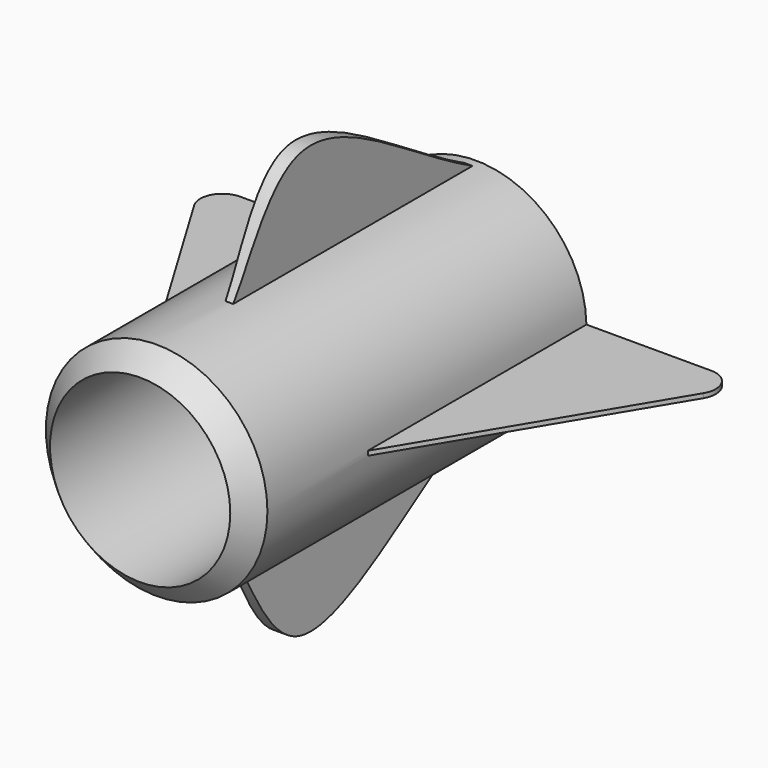
from build123d import *

# Parameters (mm, degrees)
F0_R          = 12.7
F1_DEPTH      = 50.8
F2_R          = 10.3336081204
F3_DEPTH      = 37.592
F6_DEPTH      = 0.254
F7_R          = 2.54
F9_ANGLE_BACK = 2
F9_ANGLE      = 4


# Not quite as in the source:
# - a fillet or chamfer that OpenCascade refuses, or shapes differently, is made with other operations: its cross-section is extruded or revolved along the edge and cut away or added


with BuildPart() as f1:
    # F0 (on Front) → F1 (new body)
    with BuildSketch(Plane.XZ):
        Circle(F0_R)
    extrude(amount=F1_DEPTH)

    # F2 (on face) → F3 (cut)
    with BuildSketch(Plane.XZ.offset(50.8)):
        Circle(F2_R)
    extrude(amount=-F3_DEPTH, mode=Mode.SUBTRACT)

    # F8: F6 across plane


with BuildPart() as f6:
    # F5 (on Top) → F6 (new body, symmetric)
    with BuildSketch(Plane.XY):
        Polygon((-12.446, -31.75), (-12.446, 0), (-31.496, 0), align=None)
    extrude(amount=F6_DEPTH, both=True)

    # F7
    f7_edges = [f6.edges().sort_by_distance(p)[0] for p in [
        (-31.496, 0, 0),
    ]]
    fillet(f7_edges, radius=F7_R)


with BuildPart() as f1_1:
    add(f1.part)
    add(f6.part.mirror(Plane.YZ))

    # F4 (on Right) → F9 (revolve)
    with BuildSketch(Plane.YZ, mode=Mode.PRIVATE) as f9_sk:
        with BuildLine():
            Line((0, -12.192), (-35.6481084037, -12.192))
            add(Edge.make_bspline(
                [(-35.6481084037, -12.192), (-33.4311420603, -15.1893612741), (-28.0519206857, -33.0906197841), (-9.917521665, -17.0447887187), (0, -12.192)],
                knots=[0, 0, 0, 0, 0.4167760817, 1, 1, 1, 1], degree=3))
        make_face()
    revolve(f9_sk.sketch.rotate(Axis((0, 0, 0), (0, 1, 0)), -F9_ANGLE_BACK), axis=Axis((0, 0, 0), (0, 1, 0)), revolution_arc=F9_ANGLE)

    # F10: chamfer of 5.08 on 1 edges, made by hand

    # F10_s1 → F10_t2 (revolve, cut)
    with BuildSketch(Plane.XY):
        Polygon((12.7, -45.72), (7.62, -50.8), (12.7, -50.8), align=None)
    revolve(axis=Axis((0, -50.8, 0), (0, -1, 0)), mode=Mode.SUBTRACT)



with BuildPart() as f1_2:
    add(f1_1.part)

    add(f6.part)  # F11 merges F6
    # F11: F1 across plane
    add(f1_1.part.mirror(Plane.XY))


solid = f1_2.part
